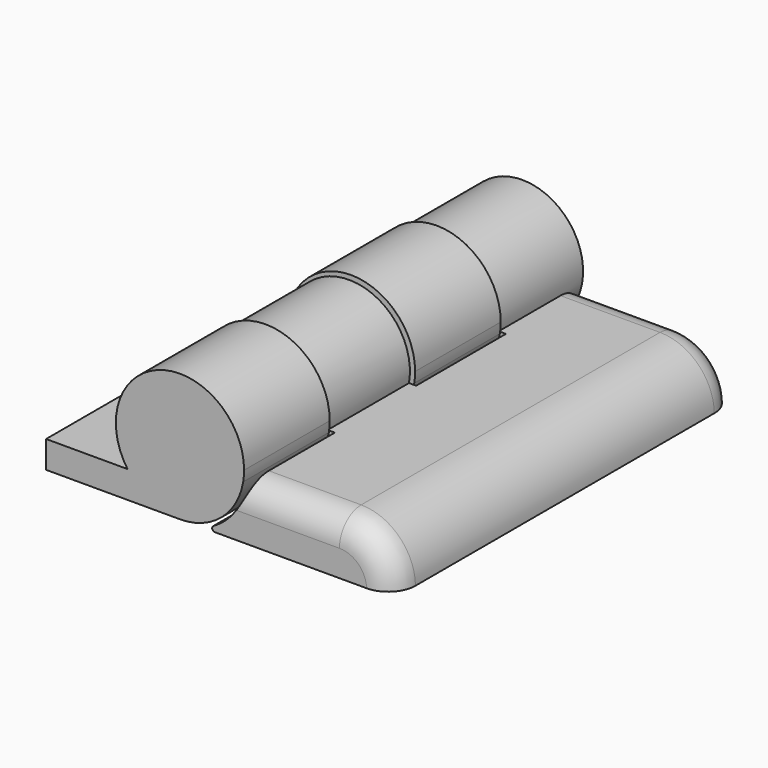
from build123d import *

# Parameters (mm, degrees)
F3_DEPTH     = 10.0076
F4_DEPTH     = 40.005
F6_START     = -19.9898
F6_DEPTH     = 10.0076
F7_DEPTH     = 10.0076
F9_START     = 20.2438
F2_R         = 3.2004
F9_DEPTH     = 9.4996
F10_DEPTH    = 10.2616
F11_START    = 20.0152
F11_DEPTH    = 9.9822
F12_START    = -19.7612
F12_DEPTH    = 11.6078
F13_DEPTH    = 9.7536
F14_T1_DEPTH = 13.1863686745
F15_T1_DEPTH = 65.405
F16_R        = 2.54


# Not quite as in the source:
# - a fillet or chamfer that OpenCascade refuses, or shapes differently, is made with other operations: its cross-section is extruded or revolved along the edge and cut away or added


with BuildPart() as f3:
    # F0 (on Front) → F3 (new body)
    with BuildSketch(Plane.XZ):
        with BuildLine():
            ThreePointArc((-4.8989745866, 2.54), (-2.7591462448, 0.6727514434), (0, 0))
            ThreePointArc((0, 0), (3.8726462994, 1.4188735822), (5.9119830007, 5.0038))
            ThreePointArc((5.9119830007, 5.0038), (5.9737602169, 5.4973887019), (5.9944, 5.9944))
            ThreePointArc((5.9944, 5.9944), (-1.8119627615, 11.7083848014), (-4.8989745866, 2.54))
        make_face()
        with BuildLine():
            ThreePointArc((-0.3048, 3.0127385839), (0, 8.9916), (0.3048, 3.0127385839))
            Line((0.3048, 3.0127385839), (0.3048, 2.808547348))
            ThreePointArc((0.3048, 2.808547348), (0, 2.794), (-0.3048, 2.808547348))
            Line((-0.3048, 2.808547348), (-0.3048, 3.0127385839))
        make_face(mode=Mode.SUBTRACT)
        with BuildLine():
            Line((-12.5189745866, 0), (0, 0))
            ThreePointArc((0, 0), (-2.7591462448, 0.6727514434), (-4.8989745866, 2.54))
            Line((-4.8989745866, 2.54), (-12.5189745866, 2.54))
            Line((-12.5189745866, 2.54), (-12.5189745866, 0))
        make_face()
    extrude(amount=-F3_DEPTH)

    # F0 (on Front) → F4 (join)
    with BuildSketch(Plane.XZ):
        with BuildLine():
            Line((0.3048, 2.808547348), (0.3048, 3.0127385839))
            ThreePointArc((0.3048, 3.0127385839), (0, 8.9916), (-0.3048, 3.0127385839))
            Line((-0.3048, 3.0127385839), (-0.3048, 2.808547348))
            ThreePointArc((-0.3048, 2.808547348), (0, 2.794), (0.3048, 2.808547348))
        make_face()
    extrude(amount=-F4_DEPTH)

    # F0 (on Front) → F6 (join)
    with BuildSketch(Plane.XZ.offset(F6_START)):
        with BuildLine():
            ThreePointArc((-4.8989745866, 2.54), (-2.7591462448, 0.6727514434), (0, 0))
            ThreePointArc((0, 0), (3.8726462994, 1.4188735822), (5.9119830007, 5.0038))
            ThreePointArc((5.9119830007, 5.0038), (5.9737602169, 5.4973887019), (5.9944, 5.9944))
            ThreePointArc((5.9944, 5.9944), (-1.8119627615, 11.7083848014), (-4.8989745866, 2.54))
        make_face()
        with BuildLine():
            ThreePointArc((-0.3048, 3.0127385839), (0, 8.9916), (0.3048, 3.0127385839))
            Line((0.3048, 3.0127385839), (0.3048, 2.808547348))
            ThreePointArc((0.3048, 2.808547348), (0, 2.794), (-0.3048, 2.808547348))
            Line((-0.3048, 2.808547348), (-0.3048, 3.0127385839))
        make_face(mode=Mode.SUBTRACT)
        with BuildLine():
            Line((-12.5189745866, 0), (0, 0))
            ThreePointArc((0, 0), (-2.7591462448, 0.6727514434), (-4.8989745866, 2.54))
            Line((-4.8989745866, 2.54), (-12.5189745866, 2.54))
            Line((-12.5189745866, 2.54), (-12.5189745866, 0))
        make_face()
    extrude(amount=-F6_DEPTH)

    # F2 (on offset) → F7 (join)
    with BuildSketch(Plane.XZ.offset(-40.005)):
        with BuildLine():
            ThreePointArc((-1.5118372742, 0.1937811178), (-3.4133287183, 1.0667211934), (-4.8989745866, 2.54))
            Line((-4.8989745866, 2.54), (-12.5189745866, 2.54))
            Line((-12.5189745866, 2.54), (-12.5189745866, 0))
            Line((-12.5189745866, 0), (-1.5366753453, 0))
            ThreePointArc((-1.5366753453, 0), (-1.4389921182, 0.0859617436), (-1.5118372742, 0.1937811178))
        make_face()
    extrude(amount=F7_DEPTH)

    # F2 (on offset) → F9 (join)
    with BuildSketch(Plane.XZ.offset(-40.005).offset(F9_START)):
        with BuildLine():
            Line((0, 0.3048), (0, 0))
            ThreePointArc((0, 0), (3.8726462994, 1.4188735822), (5.9119830007, 5.0038))
            Line((5.9119830007, 5.0038), (5.6027011164, 5.0038))
            ThreePointArc((5.6027011164, 5.0038), (-3.6561886166, 10.353738592), (0, 0.3048))
        make_face()
        with Locations((0, 5.9944)):
            Circle(F2_R, mode=Mode.SUBTRACT)
        with BuildLine():
            ThreePointArc((5.9119830007, 5.0038), (3.8726462994, 1.4188735822), (0, 0))
            Line((0, 0), (19.9898, 0))
            Line((19.9898, 0), (19.9898, 5.0038))
            Line((19.9898, 5.0038), (5.9119830007, 5.0038))
        make_face()
    extrude(amount=F9_DEPTH)

    # F0 (on Front) → F10 (join)
    with BuildSketch(Plane.XZ):
        with BuildLine():
            ThreePointArc((6.2722573002, 5.0038), (4.8747199854, 1.9250505355), (2.0951536077, 0))
            Line((2.0951536077, 0), (19.9898, 0))
            Line((19.9898, 0), (19.9898, 5.0038))
            Line((19.9898, 5.0038), (6.2722573002, 5.0038))
        make_face()
    extrude(amount=-F10_DEPTH)

    # F2 (on offset) → F11 (join)
    with BuildSketch(Plane.XZ.offset(-40.005).offset(F11_START)):
        with BuildLine():
            ThreePointArc((-1.5118372742, 0.1937811178), (-3.4133287183, 1.0667211934), (-4.8989745866, 2.54))
            Line((-4.8989745866, 2.54), (-12.5189745866, 2.54))
            Line((-12.5189745866, 2.54), (-12.5189745866, 0))
            Line((-12.5189745866, 0), (-1.5366753453, 0))
            ThreePointArc((-1.5366753453, 0), (-1.4389921182, 0.0859617436), (-1.5118372742, 0.1937811178))
        make_face()
    extrude(amount=F11_DEPTH)

    # F0 (on Front) → F12 (join)
    with BuildSketch(Plane.XZ.offset(F12_START)):
        with BuildLine():
            ThreePointArc((6.2722573002, 5.0038), (4.8747199854, 1.9250505355), (2.0951536077, 0))
            Line((2.0951536077, 0), (19.9898, 0))
            Line((19.9898, 0), (19.9898, 5.0038))
            Line((19.9898, 5.0038), (6.2722573002, 5.0038))
        make_face()
    extrude(amount=-F12_DEPTH)

    # F2 (on offset) → F13 (join)
    with BuildSketch(Plane.XZ.offset(-40.005)):
        with BuildLine():
            ThreePointArc((5.9119830007, 5.0038), (3.8726462994, 1.4188735822), (0, 0))
            Line((0, 0), (19.9898, 0))
            Line((19.9898, 0), (19.9898, 5.0038))
            Line((19.9898, 5.0038), (5.9119830007, 5.0038))
        make_face()
        with BuildLine():
            Line((0, 0.3048), (0, 0))
            ThreePointArc((0, 0), (3.8726462994, 1.4188735822), (5.9119830007, 5.0038))
            Line((5.9119830007, 5.0038), (5.6027011164, 5.0038))
            ThreePointArc((5.6027011164, 5.0038), (-3.6561886166, 10.353738592), (0, 0.3048))
        make_face()
        with Locations((0, 5.9944)):
            Circle(F2_R, mode=Mode.SUBTRACT)
    extrude(amount=F13_DEPTH)

    # F14: fillet of radius 0.254 on 1 edges, made by hand

    # F14_s2 → F14_t1 (cut)
    with BuildSketch(Plane.XZ.offset(-10.2616)):
        with BuildLine():
            ThreePointArc((3.1394818053, 0.4747846154), (3.0195052872, 0.1890511444), (3.2650610775, 0))
            Line((3.2650610775, 0), (2.0951536077, 0))
            ThreePointArc((2.0951536077, 0), (2.628061469, 0.2137605098), (3.1394818053, 0.4747846154))
        make_face()
    extrude(amount=F14_T1_DEPTH, mode=Mode.SUBTRACT)

    # F15: fillet of radius 5.08 on 1 edges, made by hand

    # F15_s2 → F15_t1 (cut)
    with BuildSketch(Plane.XZ.offset(-52.705)):
        with BuildLine():
            ThreePointArc((19.9898, -0.0762), (18.5019024484, 3.5159024484), (14.9098, 5.0038))
            Line((14.9098, 5.0038), (19.9898, 5.0038))
            Line((19.9898, 5.0038), (19.9898, -0.0762))
        make_face()
    extrude(amount=F15_T1_DEPTH, mode=Mode.SUBTRACT)

    # F16
    f16_edges = [f3.edges().sort_by_distance(p)[0] for p in [
        (10.256251, 40.005, 5.0038),
        (10.591029, 0, 5.0038),
        (18.47486, 40.005, 3.542743),
        (18.47486, 0, 3.542743),
    ]]
    fillet(f16_edges, radius=F16_R)


solid = f3.part
